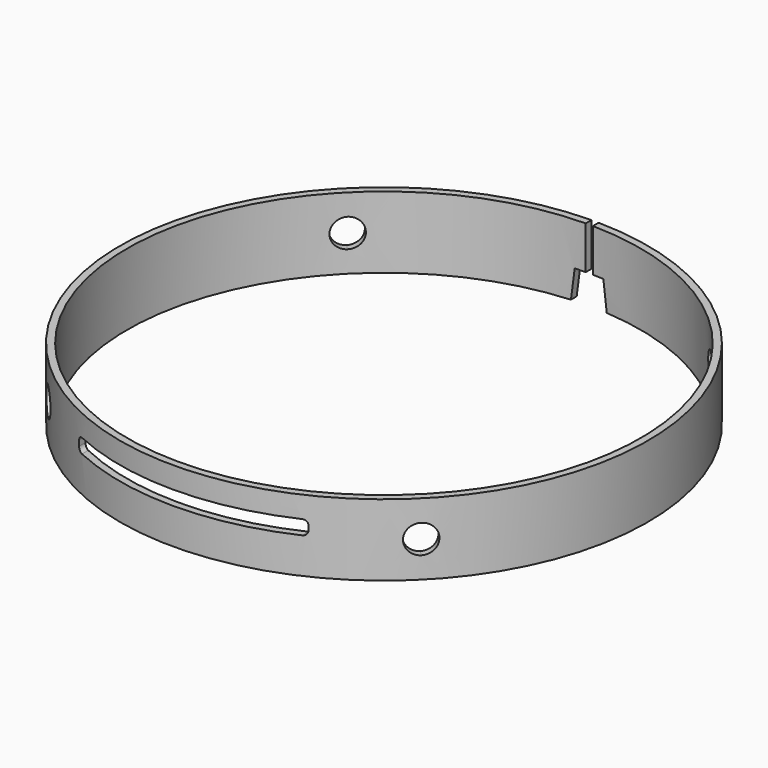
from build123d import *

# Parameters (mm, degrees)
F0_R     = 58.4999993443
F0_R_2   = 56.9124993443
F1_DEPTH = 15.875
F3_DEPTH = 62
F5_DEPTH = 61
F7_DEPTH = 80.5
F8_ANGLE = 45


# Not quite as in the source:
# - a length typed as a fraction of an inch, garbled in the dataset ("3 / 203.2 mm" for 3/8 in), is restored


with BuildPart() as f1:
    # F0 (on Top) → F1 (new body)
    with BuildSketch(Plane.XY):
        Circle(F0_R)
        Circle(F0_R_2, mode=Mode.SUBTRACT)
    extrude(amount=F1_DEPTH)

    # F2 (on Front) → F3 (cut)
    with BuildSketch(Plane.XZ):
        with BuildLine():
            Line((24.4034621794, 11.1125), (0, 11.1125))
            Line((0, 11.1125), (-24.4034621794, 11.1125))
            ThreePointArc((-24.4034621794, 11.1125), (-25.1105689606, 10.8196067812), (-25.4034621794, 10.1125))
            Line((-25.4034621794, 10.1125), (-25.4034621794, 8.9375))
            ThreePointArc((-25.4034621794, 8.9375), (-25.1105689606, 8.2303932188), (-24.4034621794, 7.9375))
            Line((-24.4034621794, 7.9375), (0, 7.9375))
            Line((0, 7.9375), (24.4034621794, 7.9375))
            ThreePointArc((24.4034621794, 7.9375), (25.1105689606, 8.2303932188), (25.4034621794, 8.9375))
            Line((25.4034621794, 8.9375), (25.4034621794, 10.1125))
            ThreePointArc((25.4034621794, 10.1125), (25.1105689606, 10.8196067812), (24.4034621794, 11.1125))
        make_face()
    extrude(amount=F3_DEPTH, mode=Mode.SUBTRACT)

    # F4 (on Front) → F5 (cut)
    with BuildSketch(Plane.XZ):
        Polygon((0, 6.35), (0, 0), (3.96875, 0), (3.175, 6.35), (0.79375, 6.35), align=None)
        Polygon((-3.96875, 0), (0, 0), (0, 6.35), (-0.79375, 6.35), (-3.175, 6.35), align=None)
        Polygon((-0.79375, 6.35), (0, 6.35), (0.79375, 6.35), (0.79375, 16.0845518112), (0, 16.0845518112), (-0.79375, 16.0845518112), align=None)
    extrude(amount=-F5_DEPTH, mode=Mode.SUBTRACT)


with BuildPart() as f7:
    # F6 (on Right) → F7 (new body, symmetric)
    with BuildSketch(Plane.YZ):
        with BuildLine():
            ThreePointArc((0, 4.7625), (2.2450640303, 5.6924359697), (3.175, 7.9375))
            ThreePointArc((3.175, 7.9375), (2.2450640303, 10.1825640303), (0, 11.1125))
            Line((0, 11.1125), (0, 4.7625))
        make_face()
        with BuildLine():
            Line((0, 4.7625), (0, 11.1125))
            ThreePointArc((0, 11.1125), (-3.175, 7.9375), (0, 4.7625))
        make_face()
    extrude(amount=F7_DEPTH, both=True)


with BuildPart() as f7_1:
    # F8: moved
    add(f7.part.rotate(Axis((0, 0, 0), (0, 0, -1)), F8_ANGLE))


with BuildPart() as f9_1:
    # F9: instance of F7
    add(f7_1.part.mirror(Plane.YZ))


with BuildPart() as f1_1:
    add(f1.part)

    # F10: cut F9_1, F7
    add(f9_1.part, mode=Mode.SUBTRACT)
    add(f7_1.part, mode=Mode.SUBTRACT)


solid = f1_1.part
